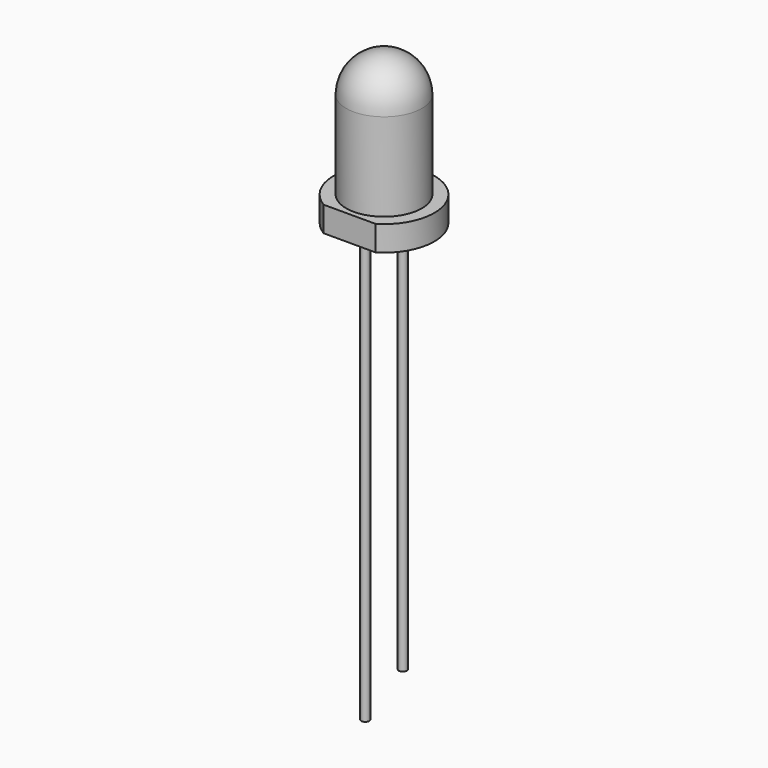
from build123d import *

# Parameters (mm, degrees)
F0_R      = 3.175
F1_DEPTH  = 1.5875
F6_W      = 20.4342100769
F6_H      = 36.2635273486
F7_DEPTH  = 10.668
F8_R      = 0.25
F9_DEPTH  = 25.4
F10_DEPTH = 26.9875


# Not quite as in the source:
# - a length typed as a fraction of an inch, garbled in the dataset ("3 / 203.2 mm" for 3/8 in), is restored


with BuildPart() as f1:
    # F0 (on Top) → F1 (new body)
    with BuildSketch(Plane.XY):
        Circle(F0_R)
    extrude(amount=F1_DEPTH)

    # F2 (on Front) → F4 (revolve)
    with BuildSketch(Plane.XZ):
        with BuildLine():
            Line((-2.3876, 0), (0, 0))
            Line((0, 0), (0, 9.525))
            ThreePointArc((0, 9.525), (-1.6882881508, 8.8256881508), (-2.3876, 7.1374))
            Line((-2.3876, 7.1374), (-2.3876, 0))
        make_face()
    revolve(axis=Axis((0, 0, 21.5854328126), (0, 0, 1)))

    # F6 (on offset) → F7 (cut)
    with BuildSketch(Plane.XZ.offset(2.7178)):
        with Locations((0.1439033076, 14.3902888522)):
            Rectangle(F6_W, F6_H)
    extrude(amount=F7_DEPTH, mode=Mode.SUBTRACT)

    # F8 (on face) → F9 (join)
    with BuildSketch(Plane(origin=(0, 0, 0), x_dir=(1, 0, 0), z_dir=(0, 0, -1))):
        with Locations((0, -1.4801331563)):
            Circle(F8_R)
        with Locations((0, 1.4801331563)):
            Circle(F8_R)
    extrude(amount=F9_DEPTH)

    # F8 (on face) → F10 (join)
    with BuildSketch(Plane(origin=(0, 0, 0), x_dir=(1, 0, 0), z_dir=(0, 0, -1))):
        with Locations((0, 1.4801331563)):
            Circle(F8_R)
    extrude(amount=F10_DEPTH)


solid = f1.part
